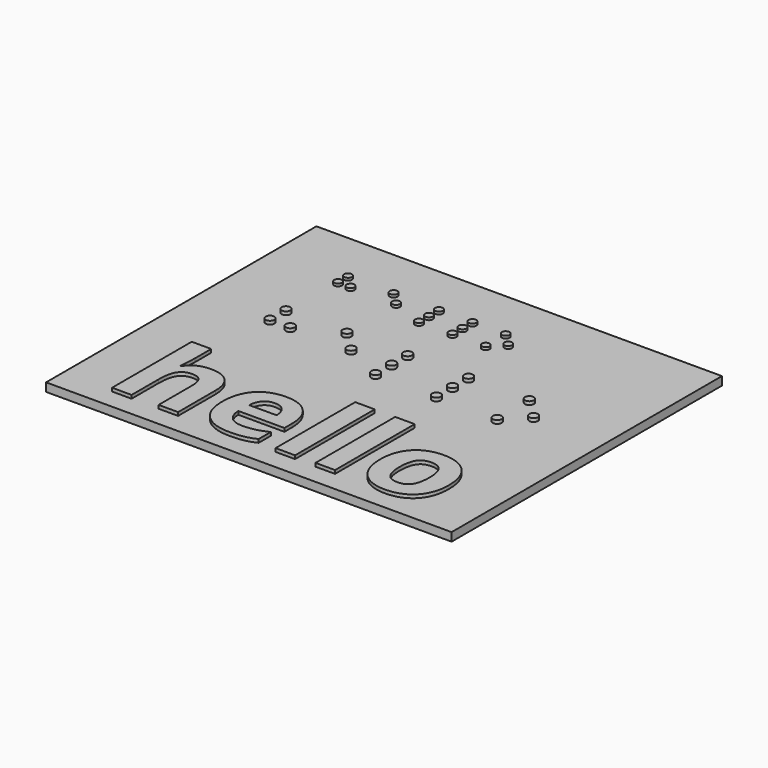
from build123d import *

# Parameters (mm, degrees)
F0_W         = 76.2
F0_H         = 63.5
F1_DEPTH     = 1.5875
F2_R         = 0.7239
F3_DEPTH     = 0.4826
F4_R         = 0.8255
F5_DEPTH     = 0.635
F6_TEXT_SIZE = 24.6153568797
F7_DEPTH     = 0.635


# Not quite as in the source:
# - Text() gives the source's letters only with a copy of the font that has no kerning and outlines rounded to 1/6400 em; it was checked with that copy


with BuildPart() as f1:
    # F0 (on Top) → F1 (new body)
    with BuildSketch(Plane.XY):
        with Locations((40.3773267701, 31.75)):
            Rectangle(F0_W, F0_H)
    extrude(amount=F1_DEPTH)

    # F2 (on face) → F3 (join)
    with BuildSketch(Plane.XY.offset(1.5875)):
        with Locations((16.2564413625, 51.114533606)):
            Circle(F2_R)
        with Locations((18.5932413625, 51.114533606)):
            Circle(F2_R)
        with Locations((16.2608381361, 53.4513294697)):
            Circle(F2_R)
        with Locations((24.82063882, 53.4513294697)):
            Circle(F2_R)
        with Locations((27.1530420464, 51.114533606)):
            Circle(F2_R)
        with Locations((33.3716452728, 48.7256667409)):
            Circle(F2_R)
        with Locations((33.3760420464, 51.0624626045)):
            Circle(F2_R)
        with Locations((33.38043882, 53.3992584682)):
            Circle(F2_R)
        with Locations((39.5946452728, 48.823941499)):
            Circle(F2_R)
        with Locations((39.5990420464, 51.1607373626)):
            Circle(F2_R)
        with Locations((39.60343882, 53.4975332263)):
            Circle(F2_R)
        with Locations((45.8176452728, 48.8574430346)):
            Circle(F2_R)
        with Locations((48.1588420464, 51.1942388983)):
            Circle(F2_R)
        with Locations((45.82643882, 53.531034762)):
            Circle(F2_R)
    extrude(amount=F3_DEPTH)

    # F4 (on face) → F5 (join)
    with BuildSketch(Plane.XY.offset(1.5875)):
        with Locations((15.9399462415, 39.2916711578)):
            Circle(F4_R)
        with Locations((15.9699697755, 35.4817894553)):
            Circle(F4_R)
        with Locations((19.7799697755, 35.4817894553)):
            Circle(F4_R)
        with Locations((27.3699462415, 39.2916711578)):
            Circle(F4_R)
        with Locations((31.2099697755, 35.4817894553)):
            Circle(F4_R)
        with Locations((38.7999462415, 39.2916711578)):
            Circle(F4_R)
        with Locations((38.8299697755, 35.4817894553)):
            Circle(F4_R)
        with Locations((38.8599933094, 31.6719077528)):
            Circle(F4_R)
        with Locations((50.2299462415, 39.2916711578)):
            Circle(F4_R)
        with Locations((50.2599697755, 35.4817894553)):
            Circle(F4_R)
        with Locations((50.2899933094, 31.6719077528)):
            Circle(F4_R)
        with Locations((61.6599462415, 39.2916711578)):
            Circle(F4_R)
        with Locations((65.4999697755, 35.4817894553)):
            Circle(F4_R)
        with Locations((61.7199933094, 31.6719077528)):
            Circle(F4_R)
    extrude(amount=F5_DEPTH)

    # F6 (on face) → F7 (join)
    with BuildSketch(Plane.XY.offset(1.5875)):
        with Locations((9.7491042688, 3.762433771)):
            Text('hello', F6_TEXT_SIZE, font='Open Sans', font_style=FontStyle.BOLD, text_align=(TextAlign.LEFT, TextAlign.BOTTOM))
    extrude(amount=F7_DEPTH)


solid = f1.part
